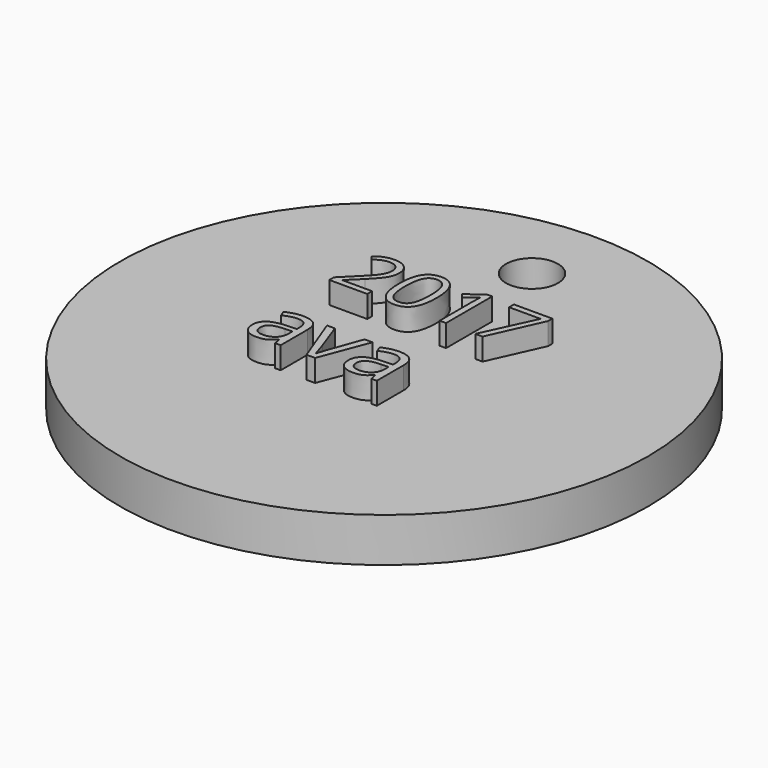
from build123d import *

# Parameters (mm, degrees)
F0_R           = 59.7896284956
F1_DEPTH       = 10
F2_R           = 5.8875647991
F3_DEPTH       = 25
F4_TEXT_SIZE   = 20.60503078
F4_TEXT_SIZE_2 = 18.3129514981
F5_DEPTH       = 5


# Not quite as in the source:
# - Text() gives the source's letters only with a copy of the font that has no kerning and outlines rounded to 1/6400 em; it was checked with that copy


with BuildPart() as f1:
    # F0 (on Top) → F1 (new body)
    with BuildSketch(Plane.XY):
        Circle(F0_R)
    extrude(amount=F1_DEPTH)

    # F2 (on face) → F3 (cut)
    with BuildSketch(Plane.XY.offset(10)):
        with Locations((0, 41.8875142932)):
            Circle(F2_R)
    extrude(amount=-F3_DEPTH, mode=Mode.SUBTRACT)

    # F4 (on face) → F5 (join)
    with BuildSketch(Plane.XY.offset(10)):
        with Locations((-21.3476847857, -14.8356221616)):
            Text('ava', F4_TEXT_SIZE, font='Open Sans', text_align=(TextAlign.LEFT, TextAlign.BOTTOM))
        with Locations((-21.3476847857, 10.0607285276)):
            Text('2017', F4_TEXT_SIZE_2, font='Open Sans', text_align=(TextAlign.LEFT, TextAlign.BOTTOM))
    extrude(amount=F5_DEPTH)


solid = f1.part
